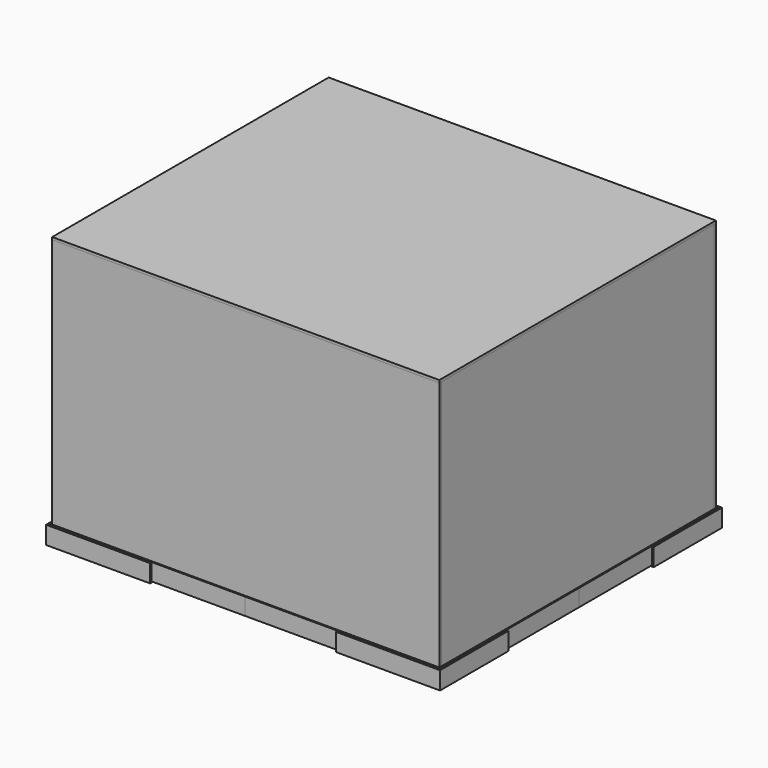
from build123d import *

# Parameters (mm, degrees)
F1_DEPTH  = 3
F2_DEPTH  = 456
F0_W      = 3
F0_H      = 305
F3_DEPTH  = 456
F4_W      = 401
F4_H      = 305
F5_DEPTH  = 3
F6_W      = 3
F6_H      = 93.4367607989
F7_DEPTH  = 10
F8_DEPTH  = 10
F6_W_2    = 109.5
F6_H_2    = 3
F6_H_3    = 1.5
F9_DEPTH  = 10
F6_W_3    = 1.5
F6_H_4    = 107.0632392011
F10_DEPTH = 10
F11_DEPTH = 10
F6_H_5    = 90.8445146084
F12_DEPTH = 10
F13_W     = 114
F13_H     = 91.9367607989
F14_DEPTH = 1
F15_DEPTH = 20


with BuildPart() as f1:
    # F0 (on Right) → F1 (new body)
    with BuildSketch(Plane.YZ):
        with BuildLine():
            Line((404, 305), (3, 305))
            Line((3, 305), (3, 0))
            Line((3, 0), (294.3445146084, 0))
            Line((294.3445146084, 0), (294.3445146084, 252.0307898521))
            ThreePointArc((294.3445146084, 252.0307898521), (302.4538769047, 260.1401521485), (310.5632392011, 252.0307898521))
            Line((310.5632392011, 252.0307898521), (310.5632392011, 0))
            Line((310.5632392011, 0), (404, 0))
            Line((404, 0), (404, 305))
        make_face()
    extrude(amount=F1_DEPTH)


with BuildPart() as f2:
    # F0 (on Right) → F2 (new body)
    with BuildSketch(Plane.YZ):
        Polygon((407, 308), (0, 308), (0, 305), (3, 305), (404, 305), (407, 305), align=None)
    extrude(amount=F2_DEPTH)


with BuildPart() as f3:
    # F0 (on Right) → F3 (new body)
    with BuildSketch(Plane.YZ):
        with Locations((1.5, 152.5)):
            Rectangle(F0_W, F0_H)
    extrude(amount=F3_DEPTH)


with BuildPart() as f3b:
    # F0 (on Right) → F3, piece 2 (new body)
    with BuildSketch(Plane.YZ):
        with Locations((405.5, 152.5)):
            Rectangle(F0_W, F0_H)
    extrude(amount=F3_DEPTH)


with BuildPart() as f5:
    # F4 (on face) → F5 (new body)
    with BuildSketch(Plane.YZ.offset(456)):
        with Locations((203.5, 152.5)):
            Rectangle(F4_W, F4_H)
    extrude(amount=-F5_DEPTH)


with BuildPart() as f7:
    # F6 (on face) → F7 (new body)
    with BuildSketch(Plane(origin=(0, 0, 0), x_dir=(1, 0, 0), z_dir=(0, 0, -1))):
        Polygon((0, -3), (0, 0), (118.5, 0), (118.5, 1.5), (-1.5, 1.5), (-1.5, -96.4367607989), (0, -96.4367607989), align=None)
        Polygon((118.5, 0), (0, 0), (0, -3), (3, -3), (118.5, -3), align=None)
        Polygon((118.5, -4.5), (118.5, -3), (3, -3), (3, -96.4367607989), (4.5, -96.4367607989), (4.5, -4.5), align=None)
        with Locations((1.5, -49.7183803995)):
            Rectangle(F6_W, F6_H)
    extrude(amount=F7_DEPTH)

    # F6 (on face) → F8, piece 4 (join)
    with BuildSketch(Plane(origin=(0, 0, 0), x_dir=(1, 0, 0), z_dir=(0, 0, -1))):
        Polygon((0, -3), (0, 0), (118.5, 0), (118.5, 1.5), (-1.5, 1.5), (-1.5, -96.4367607989), (0, -96.4367607989), align=None)
        Polygon((118.5, -4.5), (118.5, -3), (3, -3), (3, -96.4367607989), (4.5, -96.4367607989), (4.5, -4.5), align=None)
    extrude(amount=-F8_DEPTH)


with BuildPart() as f7b:
    # F6 (on face) → F7, piece 2 (new body)
    with BuildSketch(Plane(origin=(0, 0, 0), x_dir=(1, 0, 0), z_dir=(0, 0, -1))):
        Polygon((0, -407), (0, -310.5632392011), (-1.5, -310.5632392011), (-1.5, -408.5), (118.5, -408.5), (118.5, -407), align=None)
        Polygon((3, -310.5632392011), (0, -310.5632392011), (0, -407), (118.5, -407), (118.5, -404), (3, -404), align=None)
        Polygon((4.5, -310.5632392011), (3, -310.5632392011), (3, -404), (118.5, -404), (118.5, -402.5), (4.5, -402.5), align=None)
    extrude(amount=F7_DEPTH)

    # F6 (on face) → F8, piece 3 (join)
    with BuildSketch(Plane(origin=(0, 0, 0), x_dir=(1, 0, 0), z_dir=(0, 0, -1))):
        Polygon((0, -407), (0, -310.5632392011), (-1.5, -310.5632392011), (-1.5, -408.5), (118.5, -408.5), (118.5, -407), align=None)
        Polygon((4.5, -310.5632392011), (3, -310.5632392011), (3, -404), (118.5, -404), (118.5, -402.5), (4.5, -402.5), align=None)
    extrude(amount=-F8_DEPTH)


with BuildPart() as f7c:
    # F6 (on face) → F7, piece 3 (new body)
    with BuildSketch(Plane(origin=(0, 0, 0), x_dir=(1, 0, 0), z_dir=(0, 0, -1))):
        Polygon((457.5, -310.5632392011), (456, -310.5632392011), (456, -407), (337.5, -407), (337.5, -408.5), (457.5, -408.5), align=None)
        Polygon((456, -407), (456, -310.5632392011), (453, -310.5632392011), (453, -404), (337.5, -404), (337.5, -407), align=None)
        Polygon((453, -404), (453, -310.5632392011), (451.5, -310.5632392011), (451.5, -402.5), (337.5, -402.5), (337.5, -404), align=None)
    extrude(amount=F7_DEPTH)

    # F6 (on face) → F8 (join)
    with BuildSketch(Plane(origin=(0, 0, 0), x_dir=(1, 0, 0), z_dir=(0, 0, -1))):
        Polygon((457.5, -310.5632392011), (456, -310.5632392011), (456, -407), (337.5, -407), (337.5, -408.5), (457.5, -408.5), align=None)
        Polygon((453, -404), (453, -310.5632392011), (451.5, -310.5632392011), (451.5, -402.5), (337.5, -402.5), (337.5, -404), align=None)
    extrude(amount=-F8_DEPTH)


with BuildPart() as f7d:
    # F6 (on face) → F7, piece 4 (new body)
    with BuildSketch(Plane(origin=(0, 0, 0), x_dir=(1, 0, 0), z_dir=(0, 0, -1))):
        Polygon((337.5, 1.5), (337.5, 0), (456, 0), (456, -3), (456, -96.4367607989), (457.5, -96.4367607989), (457.5, 1.5), align=None)
        Polygon((456, 0), (337.5, 0), (337.5, -3), (453, -3), (456, -3), align=None)
        Polygon((453, -3), (337.5, -3), (337.5, -4.5), (451.5, -4.5), (451.5, -96.4367607989), (453, -96.4367607989), align=None)
        with Locations((454.5, -49.7183803995)):
            Rectangle(F6_W, F6_H)
    extrude(amount=F7_DEPTH)

    # F6 (on face) → F8, piece 2 (join)
    with BuildSketch(Plane(origin=(0, 0, 0), x_dir=(1, 0, 0), z_dir=(0, 0, -1))):
        Polygon((337.5, 1.5), (337.5, 0), (456, 0), (456, -3), (456, -96.4367607989), (457.5, -96.4367607989), (457.5, 1.5), align=None)
        Polygon((453, -3), (337.5, -3), (337.5, -4.5), (451.5, -4.5), (451.5, -96.4367607989), (453, -96.4367607989), align=None)
    extrude(amount=-F8_DEPTH)

    # F13 (on face) → F14 (join)
    with BuildSketch(Plane(origin=(0, 0, -10), x_dir=(1, 0, 0), z_dir=(0, 0, -1))):
        Polygon((458, 2), (458, -96.4367607989), (460, -96.4367607989), (460, 4), (337.5, 4), (337.5, 2), align=None)
        Polygon((451.5, -96.4367607989), (457.5, -96.4367607989), (457.5, 1.5), (337.5, 1.5), (337.5, -4.5), (451.5, -4.5), align=None)
        with Locations((394.5, -50.4683803995)):
            Rectangle(F13_W, F13_H)
        Polygon((457.5, 1.5), (457.5, -96.4367607989), (458, -96.4367607989), (458, 2), (337.5, 2), (337.5, 1.5), align=None)
    extrude(amount=F14_DEPTH)

    # F13 (on face) → F15 (join)
    with BuildSketch(Plane(origin=(0, 0, -10), x_dir=(1, 0, 0), z_dir=(0, 0, -1))):
        Polygon((458, 2), (458, -96.4367607989), (460, -96.4367607989), (460, 4), (337.5, 4), (337.5, 2), align=None)
    extrude(amount=-F15_DEPTH)


with BuildPart() as f9:
    # F6 (on face) → F9 (new body)
    with BuildSketch(Plane(origin=(0, 0, 0), x_dir=(1, 0, 0), z_dir=(0, 0, -1))):
        with Locations((282.75, -1.5)):
            Rectangle(F6_W_2, F6_H_2)
        with Locations((282.75, -3.75)):
            Rectangle(F6_W_2, F6_H_3)
        with Locations((282.75, 0.75)):
            Rectangle(F6_W_2, F6_H_3)
    extrude(amount=F9_DEPTH)

    # F6 (on face) → F10, piece 2 (join)
    with BuildSketch(Plane(origin=(0, 0, 0), x_dir=(1, 0, 0), z_dir=(0, 0, -1))):
        with Locations((282.75, 0.75)):
            Rectangle(F6_W_2, F6_H_3)
        with Locations((282.75, -3.75)):
            Rectangle(F6_W_2, F6_H_3)
    extrude(amount=-F10_DEPTH)


with BuildPart() as f9b:
    # F6 (on face) → F9, piece 2 (new body)
    with BuildSketch(Plane(origin=(0, 0, 0), x_dir=(1, 0, 0), z_dir=(0, 0, -1))):
        with Locations((173.25, -407.75)):
            Rectangle(F6_W_2, F6_H_3)
        with Locations((173.25, -405.5)):
            Rectangle(F6_W_2, F6_H_2)
        with Locations((173.25, -403.25)):
            Rectangle(F6_W_2, F6_H_3)
    extrude(amount=F9_DEPTH)

    # F6 (on face) → F10, piece 3 (join)
    with BuildSketch(Plane(origin=(0, 0, 0), x_dir=(1, 0, 0), z_dir=(0, 0, -1))):
        with Locations((173.25, -403.25)):
            Rectangle(F6_W_2, F6_H_3)
        with Locations((173.25, -407.75)):
            Rectangle(F6_W_2, F6_H_3)
    extrude(amount=-F10_DEPTH)


with BuildPart() as f9c:
    # F6 (on face) → F9, piece 3 (new body)
    with BuildSketch(Plane(origin=(0, 0, 0), x_dir=(1, 0, 0), z_dir=(0, 0, -1))):
        with Locations((456.75, -257.0316196005)):
            Rectangle(F6_W_3, F6_H_4)
        with Locations((454.5, -257.0316196005)):
            Rectangle(F6_W, F6_H_4)
        with Locations((452.25, -257.0316196005)):
            Rectangle(F6_W_3, F6_H_4)
    extrude(amount=F9_DEPTH)

    # F6 (on face) → F10 (join)
    with BuildSketch(Plane(origin=(0, 0, 0), x_dir=(1, 0, 0), z_dir=(0, 0, -1))):
        with Locations((456.75, -257.0316196005)):
            Rectangle(F6_W_3, F6_H_4)
        with Locations((452.25, -257.0316196005)):
            Rectangle(F6_W_3, F6_H_4)
    extrude(amount=-F10_DEPTH)


with BuildPart() as f9d:
    # F6 (on face) → F9, piece 4 (new body)
    with BuildSketch(Plane(origin=(0, 0, 0), x_dir=(1, 0, 0), z_dir=(0, 0, -1))):
        with Locations((-0.75, -149.9683803995)):
            Rectangle(F6_W_3, F6_H_4)
        with Locations((1.5, -149.9683803995)):
            Rectangle(F6_W, F6_H_4)
        with Locations((3.75, -149.9683803995)):
            Rectangle(F6_W_3, F6_H_4)
    extrude(amount=F9_DEPTH)

    # F6 (on face) → F10, piece 4 (join)
    with BuildSketch(Plane(origin=(0, 0, 0), x_dir=(1, 0, 0), z_dir=(0, 0, -1))):
        with Locations((-0.75, -149.9683803995)):
            Rectangle(F6_W_3, F6_H_4)
        with Locations((3.75, -149.9683803995)):
            Rectangle(F6_W_3, F6_H_4)
    extrude(amount=-F10_DEPTH)


with BuildPart() as f11:
    # F6 (on face) → F11 (new body)
    with BuildSketch(Plane(origin=(0, 0, 0), x_dir=(1, 0, 0), z_dir=(0, 0, -1))):
        with Locations((282.75, -407.75)):
            Rectangle(F6_W_2, F6_H_3)
        with Locations((282.75, -405.5)):
            Rectangle(F6_W_2, F6_H_2)
        with Locations((282.75, -403.25)):
            Rectangle(F6_W_2, F6_H_3)
    extrude(amount=F11_DEPTH)

    # F6 (on face) → F12, piece 2 (join)
    with BuildSketch(Plane(origin=(0, 0, 0), x_dir=(1, 0, 0), z_dir=(0, 0, -1))):
        with Locations((282.75, -407.75)):
            Rectangle(F6_W_2, F6_H_3)
        with Locations((282.75, -403.25)):
            Rectangle(F6_W_2, F6_H_3)
    extrude(amount=-F12_DEPTH)


with BuildPart() as f11b:
    # F6 (on face) → F11, piece 2 (new body)
    with BuildSketch(Plane(origin=(0, 0, 0), x_dir=(1, 0, 0), z_dir=(0, 0, -1))):
        with Locations((456.75, -149.9683803995)):
            Rectangle(F6_W_3, F6_H_4)
        with Locations((454.5, -149.9683803995)):
            Rectangle(F6_W, F6_H_4)
        with Locations((452.25, -149.9683803995)):
            Rectangle(F6_W_3, F6_H_4)
    extrude(amount=F11_DEPTH)

    # F6 (on face) → F12, piece 4 (join)
    with BuildSketch(Plane(origin=(0, 0, 0), x_dir=(1, 0, 0), z_dir=(0, 0, -1))):
        with Locations((452.25, -149.9683803995)):
            Rectangle(F6_W_3, F6_H_4)
        with Locations((456.75, -149.9683803995)):
            Rectangle(F6_W_3, F6_H_4)
    extrude(amount=-F12_DEPTH)


with BuildPart() as f11c:
    # F6 (on face) → F11, piece 3 (new body)
    with BuildSketch(Plane(origin=(0, 0, 0), x_dir=(1, 0, 0), z_dir=(0, 0, -1))):
        with Locations((173.25, 0.75)):
            Rectangle(F6_W_2, F6_H_3)
        with Locations((173.25, -1.5)):
            Rectangle(F6_W_2, F6_H_2)
        with Locations((173.25, -3.75)):
            Rectangle(F6_W_2, F6_H_3)
    extrude(amount=F11_DEPTH)

    # F6 (on face) → F12, piece 3 (join)
    with BuildSketch(Plane(origin=(0, 0, 0), x_dir=(1, 0, 0), z_dir=(0, 0, -1))):
        with Locations((173.25, -3.75)):
            Rectangle(F6_W_2, F6_H_3)
        with Locations((173.25, 0.75)):
            Rectangle(F6_W_2, F6_H_3)
    extrude(amount=-F12_DEPTH)


with BuildPart() as f11d:
    # F6 (on face) → F11, piece 4 (new body)
    with BuildSketch(Plane(origin=(0, 0, 0), x_dir=(1, 0, 0), z_dir=(0, 0, -1))):
        with Locations((3.75, -248.9222573042)):
            Rectangle(F6_W_3, F6_H_5)
        with Locations((1.5, -248.9222573042)):
            Rectangle(F6_W, F6_H_5)
        with Locations((-0.75, -248.9222573042)):
            Rectangle(F6_W_3, F6_H_5)
    extrude(amount=F11_DEPTH)

    # F6 (on face) → F12 (join)
    with BuildSketch(Plane(origin=(0, 0, 0), x_dir=(1, 0, 0), z_dir=(0, 0, -1))):
        with Locations((3.75, -248.9222573042)):
            Rectangle(F6_W_3, F6_H_5)
        with Locations((-0.75, -248.9222573042)):
            Rectangle(F6_W_3, F6_H_5)
    extrude(amount=-F12_DEPTH)


with BuildPart() as f14:
    # F13 (on face) → F14, piece 2 (new body)
    with BuildSketch(Plane(origin=(0, 0, -10), x_dir=(1, 0, 0), z_dir=(0, 0, -1))):
        with Locations((394.5, -356.5316196005)):
            Rectangle(F13_W, F13_H)
        Polygon((337.5, -408.5), (457.5, -408.5), (457.5, -310.5632392011), (451.5, -310.5632392011), (451.5, -402.5), (337.5, -402.5), align=None)
        Polygon((458, -409), (337.5, -409), (337.5, -411), (460, -411), (460, -310.5632392011), (458, -310.5632392011), align=None)
        Polygon((457.5, -310.5632392011), (457.5, -408.5), (337.5, -408.5), (337.5, -409), (458, -409), (458, -310.5632392011), align=None)
    extrude(amount=F14_DEPTH)

    # F13 (on face) → F15, piece 4 (join)
    with BuildSketch(Plane(origin=(0, 0, -10), x_dir=(1, 0, 0), z_dir=(0, 0, -1))):
        Polygon((458, -409), (337.5, -409), (337.5, -411), (460, -411), (460, -310.5632392011), (458, -310.5632392011), align=None)
    extrude(amount=-F15_DEPTH)


with BuildPart() as f14b:
    # F13 (on face) → F14, piece 3 (new body)
    with BuildSketch(Plane(origin=(0, 0, -10), x_dir=(1, 0, 0), z_dir=(0, 0, -1))):
        Polygon((118.5, -411), (118.5, -409), (-2, -409), (-2, -310.5632392011), (-4, -310.5632392011), (-4, -411), align=None)
        Polygon((118.5, -409), (118.5, -408.5), (-1.5, -408.5), (-1.5, -310.5632392011), (-2, -310.5632392011), (-2, -409), align=None)
        Polygon((-1.5, -408.5), (118.5, -408.5), (118.5, -402.5), (4.5, -402.5), (4.5, -310.5632392011), (-1.5, -310.5632392011), align=None)
        with Locations((61.5, -356.5316196005)):
            Rectangle(F13_W, F13_H)
    extrude(amount=F14_DEPTH)

    # F13 (on face) → F15, piece 3 (join)
    with BuildSketch(Plane(origin=(0, 0, -10), x_dir=(1, 0, 0), z_dir=(0, 0, -1))):
        Polygon((118.5, -411), (118.5, -409), (-2, -409), (-2, -310.5632392011), (-4, -310.5632392011), (-4, -411), align=None)
    extrude(amount=-F15_DEPTH)


with BuildPart() as f14c:
    # F13 (on face) → F14, piece 4 (new body)
    with BuildSketch(Plane(origin=(0, 0, -10), x_dir=(1, 0, 0), z_dir=(0, 0, -1))):
        Polygon((-4, -96.4367607989), (-2, -96.4367607989), (-2, 2), (118.5, 2), (118.5, 4), (-4, 4), align=None)
        Polygon((-2, -96.4367607989), (-1.5, -96.4367607989), (-1.5, 1.5), (118.5, 1.5), (118.5, 2), (-2, 2), align=None)
        Polygon((-1.5, 1.5), (-1.5, -96.4367607989), (4.5, -96.4367607989), (4.5, -4.5), (118.5, -4.5), (118.5, 1.5), align=None)
        with Locations((61.5, -50.4683803995)):
            Rectangle(F13_W, F13_H)
    extrude(amount=F14_DEPTH)

    # F13 (on face) → F15, piece 2 (join)
    with BuildSketch(Plane(origin=(0, 0, -10), x_dir=(1, 0, 0), z_dir=(0, 0, -1))):
        Polygon((-4, -96.4367607989), (-2, -96.4367607989), (-2, 2), (118.5, 2), (118.5, 4), (-4, 4), align=None)
    extrude(amount=-F15_DEPTH)


solid = Compound([f1.part, f2.part, f3.part, f3b.part, f5.part, f7.part, f7b.part, f7c.part, f7d.part, f9.part, f9b.part, f9c.part, f9d.part, f11.part, f11b.part, f11c.part, f11d.part, f14.part, f14b.part, f14c.part])
